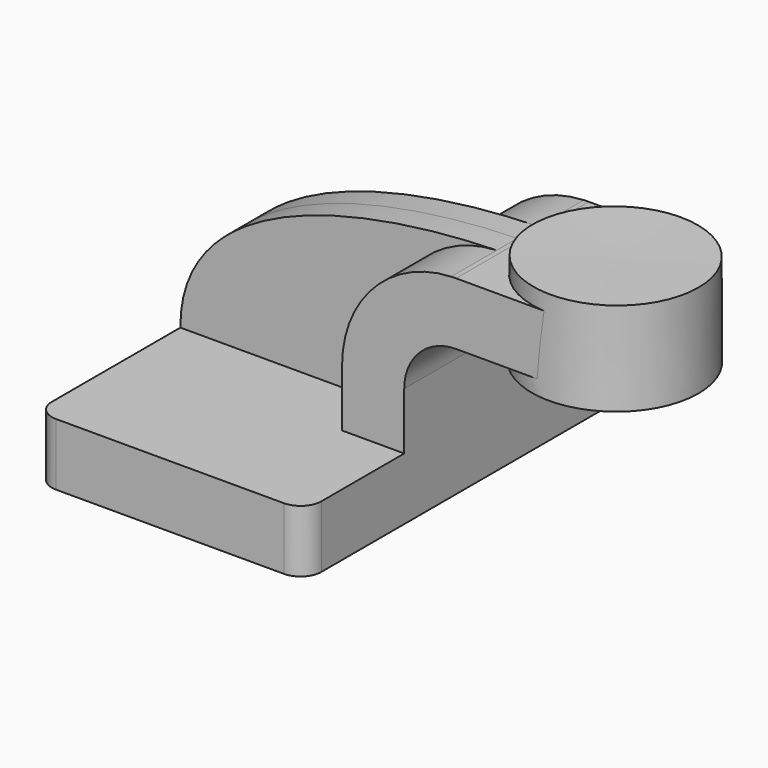
from build123d import *

# Parameters (mm, degrees)
F1_DEPTH = 63.5
F2_DEPTH = 25.4
F3_DEPTH = 7.9375
F5_R     = 6.35


with BuildPart() as f1:
    # F0 (on Front) → F1 (new body, symmetric)
    with BuildSketch(Plane.XZ):
        Polygon((-41.275, 9.525), (-41.275, -9.525), (41.275, -9.525), (41.275, 9.525), (22.225, 9.525), align=None)
    extrude(amount=F1_DEPTH, both=True)

    # F0 (on Front) → F2 (join, symmetric)
    with BuildSketch(Plane.XZ):
        Polygon((85.6770387978, 61.9252), (60.325, 61.9252), (60.325, 42.8752), (85.4846810352, 42.8752), align=None)
        with BuildLine():
            Line((22.225, 9.525), (41.275, 9.525))
            Line((41.275, 9.525), (41.275, 27.0002))
            ThreePointArc((41.275, 27.0002), (45.9246798487, 38.2255201513), (57.15, 42.8752))
            Line((57.15, 42.8752), (60.325, 42.8752))
            Line((60.325, 42.8752), (60.325, 61.9252))
            Line((60.325, 61.9252), (57.15, 61.9252))
            add(Edge.make_bspline(
                [(55.6490044481, 61.8929304371), (56.1503761632, 61.905209471), (56.6507368417, 61.9159599142), (57.15, 61.9252)],
                knots=[110.2646487764, 110.2646487764, 110.2646487764, 110.2646487764, 111.5045361635, 111.5045361635, 111.5045361635, 111.5045361635], degree=3))
            ThreePointArc((55.6490044481, 61.8929304371), (31.9291961404, 51.1593944749), (22.225, 27.0002))
            Line((22.225, 27.0002), (22.225, 9.525))
        make_face()
    extrude(amount=F2_DEPTH, both=True)

    # F0 (on Front) → F3 (join, symmetric)
    with BuildSketch(Plane.XZ):
        with BuildLine():
            add(Edge.make_bspline(
                [(-41.275, 9.525), (-41.522193166, 47.6197025146), (11.061426055, 60.8009414524), (55.6490044481, 61.8929304371)],
                knots=[0, 0, 0, 0, 110.2646487764, 110.2646487764, 110.2646487764, 110.2646487764], degree=3))
            Line((-41.275, 9.525), (22.225, 9.525))
            Line((22.225, 9.525), (22.225, 27.0002))
            ThreePointArc((22.225, 27.0002), (31.9291961404, 51.1593944749), (55.6490044481, 61.8929304371))
        make_face()
    extrude(amount=F3_DEPTH, both=True)

    # F0 (on Front) → F4 (revolve)
    with BuildSketch(Plane.XZ):
        Polygon((85.725, 66.675), (85.6770387978, 61.9252), (85.4846810352, 42.8752), (85.436463356, 38.1), (111.125, 38.1), (111.125, 66.675), align=None)
    revolve(axis=Axis((85.580731678, 0, 52.3875), (-0.0100970056, 0, -0.9999490239)))

    # F5
    f5_edges = [f1.edges().sort_by_distance(p)[0] for p in [
        (-41.275, -63.5, 0),
        (41.275, -63.5, 0),
        (41.275, 63.5, 0),
        (-41.275, 63.5, 0),
    ]]
    fillet(f5_edges, radius=F5_R)


solid = f1.part
